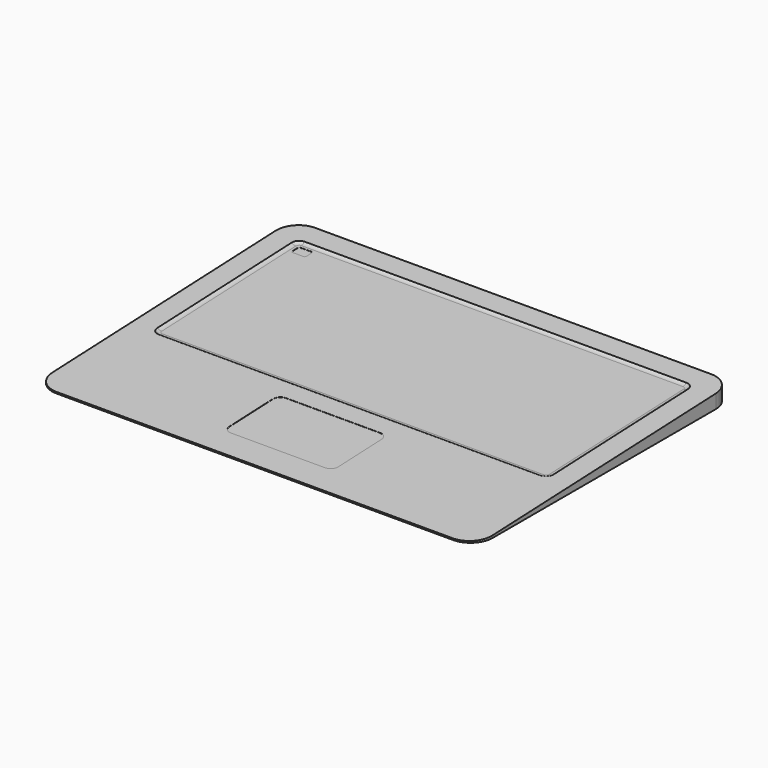
from build123d import *

# Parameters (mm, degrees)
F1_DEPTH     = 300
F2_R         = 15
F4_DEPTH     = 1
F5_T1_DEPTH  = 260
F5_T3_DEPTH  = 114.4173096389
F5_T5_DEPTH  = 114.4173096389
F5_T8_ANGLE  = 90
F5_T10_ANGLE = 90
F5_T12_ANGLE = 90
F5_T14_ANGLE = 90
F7_DEPTH     = 0.1
F9_DEPTH     = 0.1


# Not quite as in the source:
# - a fillet or chamfer that OpenCascade refuses, or shapes differently, is made with other operations: its cross-section is extruded or revolved along the edge and cut away or added


with BuildPart() as f1:
    # F0 (on Right) → F1 (new body)
    with BuildSketch(Plane.YZ):
        Polygon((-104.210527479, 1), (-104.210527479, 0), (115.789472521, 0), (115.789472521, 10), align=None)
    extrude(amount=F1_DEPTH)

    # F2
    f2_edges = [f1.edges().sort_by_distance(p)[0] for p in [
        (300, 115.789473, 5),
        (0, 115.789473, 5),
        (0, -104.210527, 0.5),
        (300, -104.210527, 0.5),
    ]]
    fillet(f2_edges, radius=F2_R)

    # F3 (on face) → F4 (cut)
    with BuildSketch(Plane(origin=(0, -0.2149512742, 5.2543644811), x_dir=(1, 0, 0), z_dir=(0, -0.040874902, 0.999164272))):
        with BuildLine():
            Line((280, 101.0889066279), (20, 101.0889066279))
            ThreePointArc((20, 101.0889066279), (16.4644660941, 99.6244405339), (15, 96.0889066279))
            Line((15, 96.0889066279), (15, -18.328403011))
            ThreePointArc((15, -18.328403011), (16.4644660941, -21.8639369169), (20, -23.328403011))
            Line((20, -23.328403011), (280, -23.328403011))
            ThreePointArc((280, -23.328403011), (283.5355339059, -21.8639369169), (285, -18.328403011))
            Line((285, -18.328403011), (285, 96.0889066279))
            ThreePointArc((285, 96.0889066279), (283.5355339059, 99.6244405339), (280, 101.0889066279))
        make_face()
    extrude(amount=-F4_DEPTH, mode=Mode.SUBTRACT)

    # F5: fillet of radius 5 on 8 edges, made by hand

    # F5_s2 → F5_t1 (join)
    with BuildSketch(Plane.YZ.offset(20)):
        with BuildLine():
            ThreePointArc((100.789472521, 9.3863636364), (99.4021842094, 8.5855726288), (97.8328546072, 8.2645746583))
            Line((97.8328546072, 8.2645746583), (100.8303474231, 8.3871993644))
            Line((100.8303474231, 8.3871993644), (100.789472521, 9.3863636364))
        make_face()
        with BuildLine():
            ThreePointArc((-23.5238580849, 4.3008182934), (-22.0757956208, 3.6160189085), (-20.485490367, 3.4242787275))
            Line((-20.485490367, 3.4242787275), (-23.4829831829, 3.3016540214))
            Line((-23.4829831829, 3.3016540214), (-23.5238580849, 4.3008182934))
        make_face()
    extrude(amount=F5_T1_DEPTH)

    # F5_s4 → F5_t3 (join)
    with BuildSketch(Plane(origin=(0, 96.0086024354, 3.9276246451), x_dir=(1, 0, 0), z_dir=(0, -0.999164272, -0.040874902))):
        with BuildLine():
            ThreePointArc((15, 5.2587593737), (16.4188611699, 4.5153428835), (18, 4.2587593737))
            Line((18, 4.2587593737), (15, 4.2587593737))
            Line((15, 4.2587593737), (15, 5.2587593737))
        make_face()
    extrude(amount=F5_T3_DEPTH)

    # F5_s6 → F5_t5 (join)
    with BuildSketch(Plane(origin=(0, -18.3130854508, -0.7491716775), x_dir=(1, 0, 0), z_dir=(0, 0.999164272, 0.040874902))):
        with BuildLine():
            ThreePointArc((285, -5.2587593737), (283.5811388301, -4.5153428835), (282, -4.2587593737))
            Line((282, -4.2587593737), (285, -4.2587593737))
            Line((285, -4.2587593737), (285, -5.2587593737))
        make_face()
    extrude(amount=F5_T5_DEPTH)

    # F5_s7 → F5_t8 (revolve)
    with BuildSketch(Plane.YZ.offset(20)):
        with BuildLine():
            ThreePointArc((100.789472521, 9.3863636364), (99.4021842094, 8.5855726288), (97.8328546072, 8.2645746583))
            Line((97.8328546072, 8.2645746583), (100.8303474231, 8.3871993644))
            Line((100.8303474231, 8.3871993644), (100.789472521, 9.3863636364))
        make_face()
    revolve(axis=Axis((20, 95.8345260632, 8.1828248542), (0, -0.040874902, 0.999164272)), revolution_arc=F5_T8_ANGLE)

    # F5_s9 → F5_t10 (revolve)
    with BuildSketch(Plane(origin=(0, -18.3130854508, -0.7491716775), x_dir=(1, 0, 0), z_dir=(0, 0.999164272, 0.040874902))):
        with BuildLine():
            ThreePointArc((15, -5.2587593737), (16.4188611699, -4.5153428835), (18, -4.2587593737))
            Line((18, -4.2587593737), (15, -4.2587593737))
            Line((15, -4.2587593737), (15, -5.2587593737))
        make_face()
    revolve(axis=Axis((20, -18.487161823, 3.5060285316), (0, -0.040874902, 0.999164272)), revolution_arc=F5_T10_ANGLE)

    # F5_s11 → F5_t12 (revolve)
    with BuildSketch(Plane.YZ.offset(280)):
        with BuildLine():
            ThreePointArc((-23.5238580849, 4.3008182934), (-22.0757956208, 3.6160189085), (-20.485490367, 3.4242787275))
            Line((-20.485490367, 3.4242787275), (-23.4829831829, 3.3016540214))
            Line((-23.4829831829, 3.3016540214), (-23.5238580849, 4.3008182934))
        make_face()
    revolve(axis=Axis((280, -18.487161823, 3.5060285316), (0, -0.040874902, 0.999164272)), revolution_arc=F5_T12_ANGLE)

    # F5_s13 → F5_t14 (revolve)
    with BuildSketch(Plane(origin=(0, 96.0086024354, 3.9276246451), x_dir=(1, 0, 0), z_dir=(0, -0.999164272, -0.040874902))):
        with BuildLine():
            ThreePointArc((285, 5.2587593737), (283.5811388301, 4.5153428835), (282, 4.2587593737))
            Line((282, 4.2587593737), (285, 4.2587593737))
            Line((285, 4.2587593737), (285, 5.2587593737))
        make_face()
    revolve(axis=Axis((280, 95.8345260632, 8.1828248542), (0, -0.040874902, 0.999164272)), revolution_arc=F5_T14_ANGLE)

    # F6 (on face) → F7 (cut)
    with BuildSketch(Plane(origin=(0, -0.2149512742, 5.2543644811), x_dir=(1, 0, 0), z_dir=(0, -0.040874902, 0.999164272))):
        with BuildLine():
            Line((182.0928883553, -37.4153330922), (117.9071116447, -37.4153330922))
            ThreePointArc((117.9071116447, -37.4153330922), (114.3715777388, -38.8797991863), (112.9071116447, -42.4153330922))
            Line((112.9071116447, -42.4153330922), (112.9071116447, -79.291882813))
            ThreePointArc((112.9071116447, -79.291882813), (114.3715777388, -82.8274167189), (117.9071116447, -84.291882813))
            Line((117.9071116447, -84.291882813), (182.0928883553, -84.291882813))
            ThreePointArc((182.0928883553, -84.291882813), (185.6284222612, -82.8274167189), (187.0928883553, -79.291882813))
            Line((187.0928883553, -79.291882813), (187.0928883553, -42.4153330922))
            ThreePointArc((187.0928883553, -42.4153330922), (185.6284222612, -38.8797991863), (182.0928883553, -37.4153330922))
        make_face()
    extrude(amount=-F7_DEPTH, mode=Mode.SUBTRACT)

    # F8 (on face) → F9 (cut)
    with BuildSketch(Plane(origin=(0, -0.1740763722, 4.2552002091), x_dir=(1, 0, 0), z_dir=(0, -0.040874902, 0.999164272))):
        with BuildLine():
            Line((28.5042302459, 96.0889066279), (21, 96.0889066279))
            ThreePointArc((21, 96.0889066279), (20.2928932188, 95.7960134091), (20, 95.0889066279))
            Line((20, 95.0889066279), (20, 90.473426342))
            ThreePointArc((20, 90.473426342), (20.2928932188, 89.7663195608), (21, 89.473426342))
            Line((21, 89.473426342), (28.5042302459, 89.473426342))
            ThreePointArc((28.5042302459, 89.473426342), (29.2113370271, 89.7663195608), (29.5042302459, 90.473426342))
            Line((29.5042302459, 90.473426342), (29.5042302459, 95.0889066279))
            ThreePointArc((29.5042302459, 95.0889066279), (29.2113370271, 95.7960134091), (28.5042302459, 96.0889066279))
        make_face()
    extrude(amount=-F9_DEPTH, mode=Mode.SUBTRACT)


solid = f1.part
